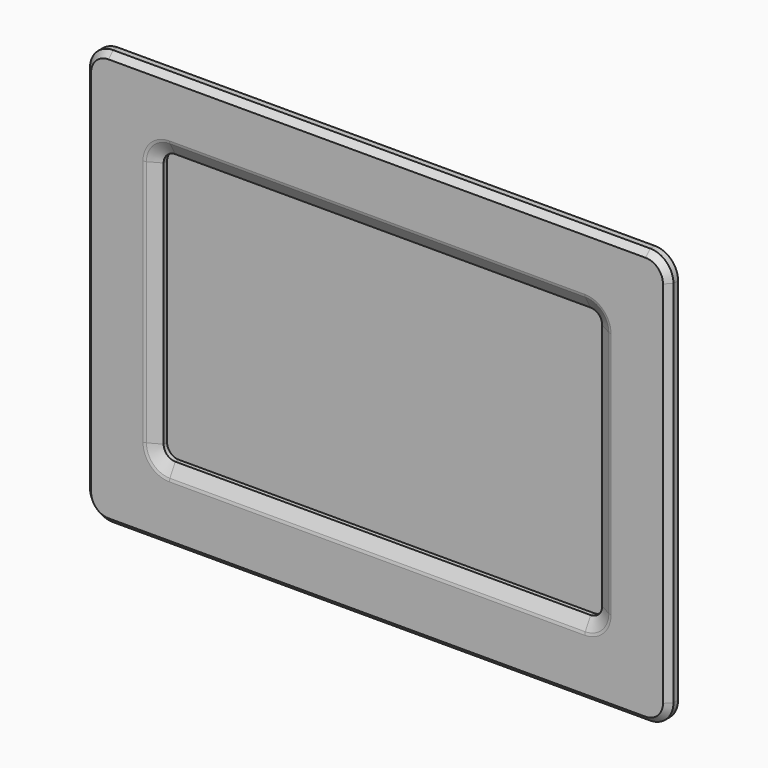
from build123d import *

# Parameters (mm, degrees)
F0_W         = 151.2998556506
F0_H         = 93.3873314755
F1_DEPTH     = 0.5
F3_DEPTH     = 4
F4_SIZE2     = 2.54
F4_SIZE      = 4.572
F5_T1_DEPTH  = 85.3873314755
F5_T3_DEPTH  = 143.2998556506
F5_T5_DEPTH  = 185.2998556506
F5_T7_DEPTH  = 127.3873314755
F5_T10_ANGLE = 90
F5_T12_ANGLE = 90
F5_T14_ANGLE = 90
F5_T16_ANGLE = 90
F5_T18_ANGLE = 90
F5_T20_ANGLE = 90
F5_T22_ANGLE = 90
F5_T24_ANGLE = 90
F7_DEPTH     = 1.5
F8_W         = 171.2998556506
F8_H         = 113.3873314755
F9_DEPTH     = 12
F10_R        = 2


# Not quite as in the source:
# - a fillet or chamfer that OpenCascade refuses, or shapes differently, is made with other operations: its cross-section is extruded or revolved along the edge and cut away or added


with BuildPart() as f1:
    # F0 (on Front) → F1 (new body)
    with BuildSketch(Plane.XZ):
        Rectangle(F0_W, F0_H)
    extrude(amount=F1_DEPTH)


with BuildPart() as f3:
    # F2 (on face) → F3 (new body)
    with BuildSketch(Plane.XZ.offset(0.5)):
        with BuildLine():
            ThreePointArc((-100.6499278253, -63.6936657378), (-98.3067820748, -69.3505199872), (-92.6499278253, -71.6936657378))
            Line((-92.6499278253, -71.6936657378), (92.6499278253, -71.6936657378))
            ThreePointArc((92.6499278253, -71.6936657378), (98.3067820748, -69.3505199872), (100.6499278253, -63.6936657378))
            Line((100.6499278253, -63.6936657378), (100.6499278253, 63.6936657378))
            ThreePointArc((100.6499278253, 63.6936657378), (98.3067820748, 69.3505199872), (92.6499278253, 71.6936657378))
            Line((92.6499278253, 71.6936657378), (-92.6499278253, 71.6936657378))
            ThreePointArc((-92.6499278253, 71.6936657378), (-98.3067820748, 69.3505199872), (-100.6499278253, 63.6936657378))
            Line((-100.6499278253, 63.6936657378), (-100.6499278253, -63.6936657378))
        make_face()
        Polygon((71.6499278253, -46.6936657378), (-71.6499278253, -46.6936657378), (-75.6499278253, -46.6936657378), (-75.6499278253, -42.6936657378), (-75.6499278253, 42.6936657378), (-75.6499278253, 46.6936657378), (-71.6499278253, 46.6936657378), (71.6499278253, 46.6936657378), (75.6499278253, 46.6936657378), (75.6499278253, 42.6936657378), (75.6499278253, -42.6936657378), (75.6499278253, -46.6936657378), align=None, mode=Mode.SUBTRACT)
        with BuildLine():
            ThreePointArc((71.6499278253, 46.6936657378), (74.47835495, 45.5220928625), (75.6499278253, 42.6936657378))
            Line((75.6499278253, 42.6936657378), (75.6499278253, 46.6936657378))
            Line((75.6499278253, 46.6936657378), (71.6499278253, 46.6936657378))
        make_face()
        with BuildLine():
            Line((-75.6499278253, -46.6936657378), (-71.6499278253, -46.6936657378))
            ThreePointArc((-71.6499278253, -46.6936657378), (-74.47835495, -45.5220928625), (-75.6499278253, -42.6936657378))
            Line((-75.6499278253, -42.6936657378), (-75.6499278253, -46.6936657378))
        make_face()
        with BuildLine():
            ThreePointArc((75.6499278253, -42.6936657378), (74.47835495, -45.5220928625), (71.6499278253, -46.6936657378))
            Line((71.6499278253, -46.6936657378), (75.6499278253, -46.6936657378))
            Line((75.6499278253, -46.6936657378), (75.6499278253, -42.6936657378))
        make_face()
        with BuildLine():
            Line((-75.6499278253, 46.6936657378), (-75.6499278253, 42.6936657378))
            ThreePointArc((-75.6499278253, 42.6936657378), (-74.47835495, 45.5220928625), (-71.6499278253, 46.6936657378))
            Line((-71.6499278253, 46.6936657378), (-75.6499278253, 46.6936657378))
        make_face()
    extrude(amount=F3_DEPTH)

    # F4
    f4_edges = [f3.edges().sort_by_distance(p)[0] for p in [
        (-75.649928, -4.5, 0),
    ]]
    f4_side = f3.faces().sort_by_distance((-96.55919, -4.5, -67.602928))[0]
    chamfer(f4_edges, length=F4_SIZE, length2=F4_SIZE2, reference=f4_side)

    # F5: chamfer of 2 on 16 edges, made by hand

    # F5_s2 → F5_t1 (cut)
    with BuildSketch(Plane.XY.offset(-42.6936657378)):
        Polygon((-79.7688940193, -4.2483145522), (-80.7401798817, -4.5), (-80.2219278253, -4.5), align=None)
        Polygon((80.7401798817, -4.5), (79.7688940193, -4.2483145522), (80.2219278253, -4.5), align=None)
    extrude(amount=F5_T1_DEPTH, mode=Mode.SUBTRACT)

    # F5_s4 → F5_t3 (cut)
    with BuildSketch(Plane.YZ.offset(-71.6499278253)):
        Polygon((-4.5, -51.7839177941), (-4.2483145522, -50.8126319318), (-4.5, -51.2656657378), align=None)
        Polygon((-4.5, 51.7839177941), (-4.2483145522, 50.8126319318), (-4.5, 51.2656657378), align=None)
    extrude(amount=F5_T3_DEPTH, mode=Mode.SUBTRACT)

    # F5_s6 → F5_t5 (cut)
    with BuildSketch(Plane.YZ.offset(-92.6499278253)):
        Polygon((-4.5, -69.6936657378), (-2.5, -71.6936657378), (-4.5, -71.6936657378), align=None)
        Polygon((-4.5, 69.6936657378), (-2.5, 71.6936657378), (-4.5, 71.6936657378), align=None)
    extrude(amount=F5_T5_DEPTH, mode=Mode.SUBTRACT)

    # F5_s8 → F5_t7 (cut)
    with BuildSketch(Plane.XY.offset(-63.6936657378)):
        Polygon((98.6499278253, -4.5), (100.6499278253, -2.5), (100.6499278253, -4.5), align=None)
        Polygon((-98.6499278253, -4.5), (-100.6499278253, -2.5), (-100.6499278253, -4.5), align=None)
    extrude(amount=F5_T7_DEPTH, mode=Mode.SUBTRACT)

    # F5_s9 → F5_t10 (revolve, cut)
    with BuildSketch(Plane.YZ.offset(-71.6499278253)):
        Polygon((-4.2483145522, -50.8126319318), (-4.5, -51.7839177941), (-4.5, -51.2656657378), align=None)
    revolve(axis=Axis((-71.6499278253, -4.5, -42.6936657378), (0, 1, 0)), revolution_arc=F5_T10_ANGLE, mode=Mode.SUBTRACT)

    # F5_s11 → F5_t12 (revolve, cut)
    with BuildSketch(Plane.XY.offset(42.6936657378)):
        Polygon((-80.7401798817, -4.5), (-79.7688940193, -4.2483145522), (-80.2219278253, -4.5), align=None)
    revolve(axis=Axis((-71.6499278253, -4.5, 42.6936657378), (0, 1, 0)), revolution_arc=F5_T12_ANGLE, mode=Mode.SUBTRACT)

    # F5_s13 → F5_t14 (revolve, cut)
    with BuildSketch(Plane.XY.offset(-42.6936657378)):
        Polygon((80.7401798817, -4.5), (79.7688940193, -4.2483145522), (80.2219278253, -4.5), align=None)
    revolve(axis=Axis((71.6499278253, -4.5, -42.6936657378), (0, 1, 0)), revolution_arc=F5_T14_ANGLE, mode=Mode.SUBTRACT)

    # F5_s15 → F5_t16 (revolve, cut)
    with BuildSketch(Plane.YZ.offset(71.6499278253)):
        Polygon((-4.5, 51.7839177941), (-4.2483145522, 50.8126319318), (-4.5, 51.2656657378), align=None)
    revolve(axis=Axis((71.6499278253, -4.5, 42.6936657378), (0, 1, 0)), revolution_arc=F5_T16_ANGLE, mode=Mode.SUBTRACT)

    # F5_s17 → F5_t18 (revolve, cut)
    with BuildSketch(Plane.XY.offset(-63.6936657378)):
        Polygon((-98.6499278253, -4.5), (-100.6499278253, -2.5), (-100.6499278253, -4.5), align=None)
    revolve(axis=Axis((-92.6499278253, -4.5, -63.6936657378), (0, -1, 0)), revolution_arc=F5_T18_ANGLE, mode=Mode.SUBTRACT)

    # F5_s19 → F5_t20 (revolve, cut)
    with BuildSketch(Plane.YZ.offset(92.6499278253)):
        Polygon((-4.5, -69.6936657378), (-2.5, -71.6936657378), (-4.5, -71.6936657378), align=None)
    revolve(axis=Axis((92.6499278253, -4.5, -63.6936657378), (0, -1, 0)), revolution_arc=F5_T20_ANGLE, mode=Mode.SUBTRACT)

    # F5_s21 → F5_t22 (revolve, cut)
    with BuildSketch(Plane.XY.offset(63.6936657378)):
        Polygon((98.6499278253, -4.5), (100.6499278253, -2.5), (100.6499278253, -4.5), align=None)
    revolve(axis=Axis((92.6499278253, -4.5, 63.6936657378), (0, -1, 0)), revolution_arc=F5_T22_ANGLE, mode=Mode.SUBTRACT)

    # F5_s23 → F5_t24 (revolve, cut)
    with BuildSketch(Plane.YZ.offset(-92.6499278253)):
        Polygon((-4.5, 69.6936657378), (-2.5, 71.6936657378), (-4.5, 71.6936657378), align=None)
    revolve(axis=Axis((-92.6499278253, -4.5, 63.6936657378), (0, -1, 0)), revolution_arc=F5_T24_ANGLE, mode=Mode.SUBTRACT)


with BuildPart() as f7:
    # F6 (on face) → F7 (new body)
    with BuildSketch(Plane(origin=(0, -0.5, 0), x_dir=(-1, 0, 0), z_dir=(0, 1, 0))):
        with BuildLine():
            Line((98.1499278253, -63.6936657378), (98.1499278253, 63.6936657378))
            ThreePointArc((98.1499278253, 63.6936657378), (96.5390151218, 67.5827530343), (92.6499278253, 69.1936657378))
            Line((92.6499278253, 69.1936657378), (-92.6499278253, 69.1936657378))
            ThreePointArc((-92.6499278253, 69.1936657378), (-96.5390151218, 67.5827530343), (-98.1499278253, 63.6936657378))
            Line((-98.1499278253, 63.6936657378), (-98.1499278253, -63.6936657378))
            ThreePointArc((-98.1499278253, -63.6936657378), (-96.5390151218, -67.5827530343), (-92.6499278253, -69.1936657378))
            Line((-92.6499278253, -69.1936657378), (92.6499278253, -69.1936657378))
            ThreePointArc((92.6499278253, -69.1936657378), (96.5390151218, -67.5827530343), (98.1499278253, -63.6936657378))
        make_face()
        with BuildLine():
            Line((-92.1499278253, 65.1936657378), (92.1499278253, 65.1936657378))
            ThreePointArc((92.1499278253, 65.1936657378), (93.5641413877, 64.6078793001), (94.1499278253, 63.1936657378))
            Line((94.1499278253, 63.1936657378), (94.1499278253, -63.1936657378))
            ThreePointArc((94.1499278253, -63.1936657378), (93.5641413877, -64.6078793001), (92.1499278253, -65.1936657378))
            Line((92.1499278253, -65.1936657378), (-92.1499278253, -65.1936657378))
            ThreePointArc((-92.1499278253, -65.1936657378), (-93.5641413877, -64.6078793001), (-94.1499278253, -63.1936657378))
            Line((-94.1499278253, -63.1936657378), (-94.1499278253, 63.1936657378))
            ThreePointArc((-94.1499278253, 63.1936657378), (-93.5641413877, 64.6078793001), (-92.1499278253, 65.1936657378))
        make_face(mode=Mode.SUBTRACT)
    extrude(amount=F7_DEPTH)


with BuildPart() as f9:
    # F8 (on face) → F9 (new body)
    with BuildSketch(Plane(origin=(0, -0.5, 0), x_dir=(-1, 0, 0), z_dir=(0, 1, 0))):
        Rectangle(F8_W, F8_H)
    extrude(amount=F9_DEPTH)

    # F10
    f10_edges = [f9.edges().sort_by_distance(p)[0] for p in [
        (0, 11.5, 56.693666),
        (-85.649928, 11.5, 0),
        (-85.649928, 5.5, 56.693666),
        (85.649928, 5.5, 56.693666),
        (85.649928, 11.5, 0),
        (85.649928, 5.5, -56.693666),
        (0, 11.5, -56.693666),
        (-85.649928, 5.5, -56.693666),
    ]]
    fillet(f10_edges, radius=F10_R)


solid = Compound([f1.part, f3.part, f7.part, f9.part])
